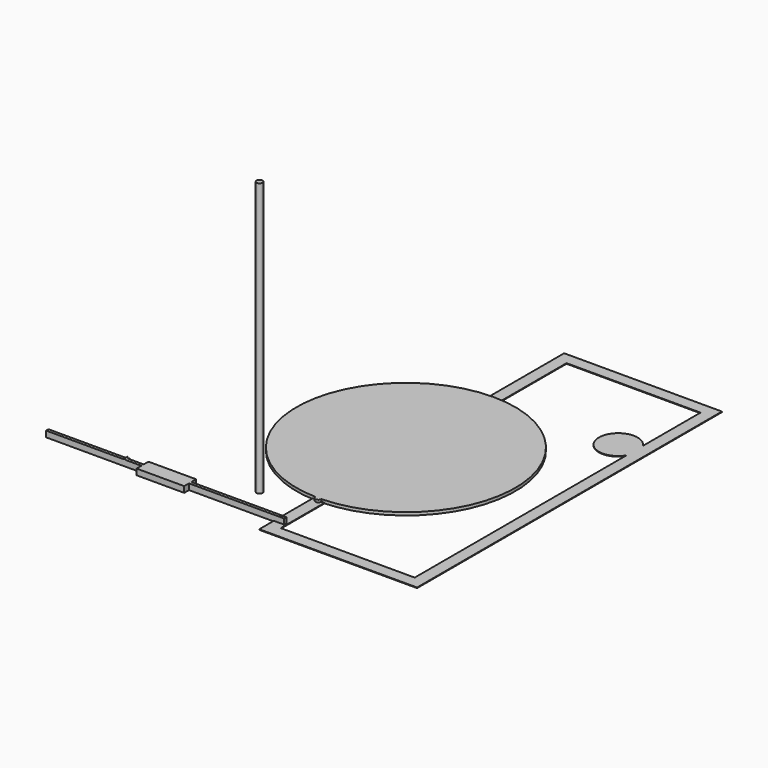
from build123d import *

# Parameters (mm, degrees)
F0_W      = 1016
F0_H      = 12.7
F0_R      = 3.175
F1_DEPTH  = 25.4
F2_R      = 6.35
F3_DEPTH  = 12.7
F5_DEPTH  = 12.7
F6_R      = 12.7
F7_DEPTH  = 1165.225
F9_DEPTH  = 12.7
F10_W     = 203.2
F10_H     = 25.4
F11_DEPTH = 25.4
F12_W     = 571.5
F12_H     = 50.8
F13_DEPTH = 2.54


# Not quite as in the source:
# - a pattern or mirror of a feature is missing from the dataset's text; its kind, count and spacing are read off the source's solid


with BuildPart() as f1:
    # F0 (on Top) → F1 (new body)
    with BuildSketch(Plane.XY):
        with Locations((-488.95, 0)):
            Rectangle(F0_W, F0_H)
        Circle(F0_R, mode=Mode.SUBTRACT)
    extrude(amount=F1_DEPTH)

    # F2 (on face) → F3 (join)
    with BuildSketch(Plane(origin=(0, 6.35, 0), x_dir=(-1, 0, 0), z_dir=(0, 1, 0))):
        with Locations((660.4, 12.7)):
            Circle(F2_R)
    extrude(amount=F3_DEPTH)

    # F8 (on face) → F9 (join)
    with BuildSketch(Plane.XZ.offset(6.35)):
        with BuildLine():
            ThreePointArc((-660.4, 31.75), (-662.2598719395, 27.2598719395), (-666.75, 25.4))
            Line((-666.75, 25.4), (-654.05, 25.4))
            ThreePointArc((-654.05, 25.4), (-658.5401280605, 27.2598719395), (-660.4, 31.75))
        make_face()
    extrude(amount=-F9_DEPTH)

    # F10 (on face) → F11 (join)
    with BuildSketch(Plane.XZ.offset(6.35)):
        with Locations((-488.95, 12.7)):
            Rectangle(F10_W, F10_H)
    f11 = extrude(amount=F11_DEPTH)

    # F11_copies: F11 across plane
    add(f11.mirror(Plane.ZX))


with BuildPart() as f5:
    # F4 (on Top) → F5 (new body)
    with BuildSketch(Plane.XY):
        with BuildLine():
            ThreePointArc((-12.6988245094, 199.7835319932), (0, 186.9107428776), (12.6988245094, 199.7835319932))
            ThreePointArc((12.6988245094, 199.7835319932), (0, 1133.0607428776), (-12.6988245094, 199.7835319932))
        make_face()
    extrude(amount=F5_DEPTH)


with BuildPart() as f7:
    # F6 (on Top) → F7 (new body)
    with BuildSketch(Plane.XY):
        with Locations((-195.9813982248, 130.7074129581)):
            Circle(F6_R)
    extrude(amount=F7_DEPTH)


with BuildPart() as f13:
    # F12 (on Top) → F13 (new body)
    with BuildSketch(Plane.XY):
        Polygon((-25.4, -83.82), (25.4, -83.82), (25.4, -33.02), (25.4, 1490.98), (25.4, 1541.78), (-25.4, 1541.78), align=None)
        with Locations((311.15, 1516.38)):
            Rectangle(F12_W, F12_H)
        with BuildLine():
            Line((596.9, -33.02), (596.9, -83.82))
            Line((596.9, -83.82), (647.7, -83.82))
            Line((647.7, -83.82), (647.7, 1541.78))
            Line((647.7, 1541.78), (596.9, 1541.78))
            Line((596.9, 1541.78), (596.9, 1490.98))
            Line((596.9, 1490.98), (596.9, 1183.8190905123))
            ThreePointArc((596.9, 1183.8190905123), (606.3614745797, 1162.7202505992), (609.6, 1139.825))
            ThreePointArc((609.6, 1139.825), (606.3614745797, 1116.9297494008), (596.9, 1095.8309094877))
            Line((596.9, 1095.8309094877), (596.9, -33.02))
        make_face()
        with BuildLine():
            ThreePointArc((596.9, 1183.8190905123), (444.5, 1139.825), (596.9, 1095.8309094877))
            Line((596.9, 1095.8309094877), (596.9, 1183.8190905123))
        make_face()
        with BuildLine():
            Line((596.9, 1183.8190905123), (596.9, 1095.8309094877))
            ThreePointArc((596.9, 1095.8309094877), (606.3614745797, 1116.9297494008), (609.6, 1139.825))
            ThreePointArc((609.6, 1139.825), (606.3614745797, 1162.7202505992), (596.9, 1183.8190905123))
        make_face()
        with Locations((311.15, -58.42)):
            Rectangle(F12_W, F12_H)
    extrude(amount=F13_DEPTH)


solid = Compound([f1.part, f5.part, f7.part, f13.part])
